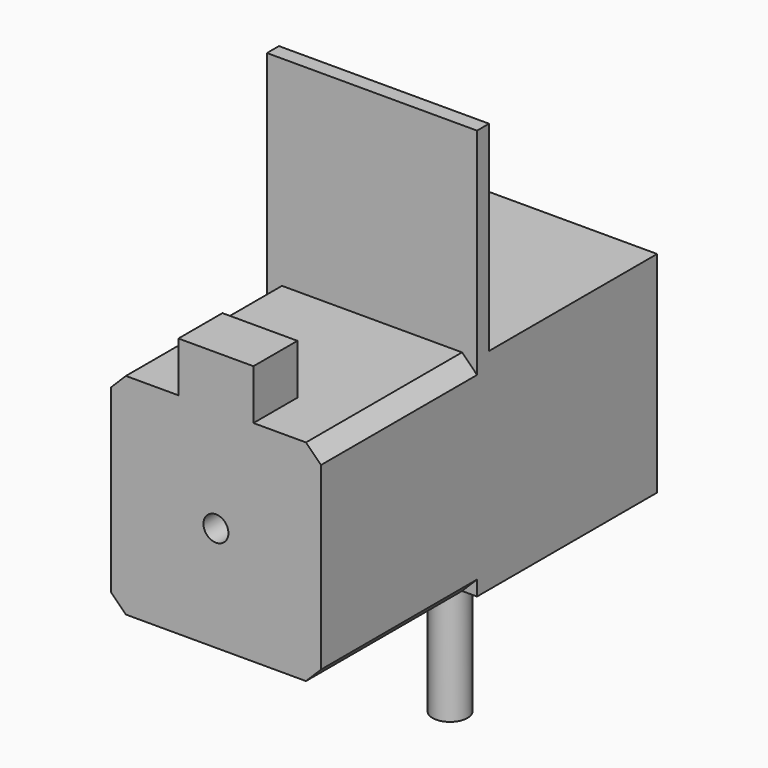
from build123d import *

# Parameters (mm, degrees)
F0_W      = 42
F0_H      = 42
F0_R      = 1.25
F0_R_2    = 11
F0_R_3    = 4.5
F0_R_4    = 2.5
F1_DEPTH  = 39
F2_SIZE   = 3
F3_DEPTH  = 2
F5_W      = 15
F5_H      = 11
F6_DEPTH  = 10
F7_DEPTH  = 45
F8_W      = 42
F8_H      = 3
F9_DEPTH  = 40
F11_DEPTH = 30


# Not quite as in the source:
# - the program builds the solid bodies; features that only make, move or delete a surface that nothing else refers to are left out


with BuildPart() as f1:
    # F0 (on Front) → F1 (new body)
    with BuildSketch(Plane.XZ):
        with Locations((-22.9883964362, 22.6771618161)):
            Rectangle(F0_W, F0_H)
        with Locations((-38.4247341791, 7.1771618161)):
            Circle(F0_R, mode=Mode.SUBTRACT)
        with Locations((-7.4883964362, 7.1771618161)):
            Circle(F0_R, mode=Mode.SUBTRACT)
        with Locations((-38.4247341791, 38.1764436699)):
            Circle(F0_R, mode=Mode.SUBTRACT)
        with Locations((-22.9883964362, 22.6771618161)):
            Circle(F0_R_2, mode=Mode.SUBTRACT)
        with Locations((-7.4883964362, 38.1778829577)):
            Circle(F0_R, mode=Mode.SUBTRACT)
        with Locations((-22.9883964362, 22.6771618161)):
            Circle(F0_R_2)
        with Locations((-22.9883964362, 22.6771618161)):
            Circle(F0_R_3, mode=Mode.SUBTRACT)
        with Locations((-22.9883964362, 22.6771618161)):
            Circle(F0_R_3)
        with Locations((-22.9883964362, 22.6771618161)):
            Circle(F0_R_4, mode=Mode.SUBTRACT)
        with Locations((-38.4247341791, 38.1764436699)):
            Circle(F0_R)
        with Locations((-7.4883964362, 7.1771618161)):
            Circle(F0_R)
        with Locations((-38.4247341791, 7.1771618161)):
            Circle(F0_R)
        with Locations((-7.4883964362, 38.1778829577)):
            Circle(F0_R)
    extrude(amount=F1_DEPTH)

    # F2
    f2_edges = [f1.edges().sort_by_distance(p)[0] for p in [
        (-43.988396, -19.5, 1.677162),
        (-1.988396, -19.5, 1.677162),
        (-1.988396, -19.5, 43.677162),
        (-43.988396, -19.5, 43.677162),
    ]]
    chamfer(f2_edges, length=F2_SIZE)

    # F0 (on Front) → F3 (join)
    with BuildSketch(Plane.XZ):
        with Locations((-22.9883964362, 22.6771618161)):
            Circle(F0_R_2)
        with Locations((-22.9883964362, 22.6771618161)):
            Circle(F0_R_3, mode=Mode.SUBTRACT)
    extrude(amount=-F3_DEPTH)

    # F5 (on face) → F6 (join)
    with BuildSketch(Plane.XY.offset(43.6771618161)):
        with Locations((-22.9883964362, -33.5)):
            Rectangle(F5_W, F5_H)
    extrude(amount=F6_DEPTH)

    # F0 (on Front) → F7 (join)
    with BuildSketch(Plane.XZ):
        with Locations((-22.9883964362, 22.6771618161)):
            Rectangle(F0_W, F0_H)
        with Locations((-38.4247341791, 7.1771618161)):
            Circle(F0_R, mode=Mode.SUBTRACT)
        with Locations((-7.4883964362, 7.1771618161)):
            Circle(F0_R, mode=Mode.SUBTRACT)
        with Locations((-38.4247341791, 38.1764436699)):
            Circle(F0_R, mode=Mode.SUBTRACT)
        with Locations((-22.9883964362, 22.6771618161)):
            Circle(F0_R_2, mode=Mode.SUBTRACT)
        with Locations((-7.4883964362, 38.1778829577)):
            Circle(F0_R, mode=Mode.SUBTRACT)
    extrude(amount=-F7_DEPTH)

    # F8 (on face) → F9 (join)
    with BuildSketch(Plane.XY.offset(43.6771618161)):
        with Locations((-22.9883964362, 1.5)):
            Rectangle(F8_W, F8_H)
    extrude(amount=F9_DEPTH)


with BuildPart() as f11:
    # F10 (on face) → F11 (new body)
    with BuildSketch(Plane(origin=(0, 0, 1.6771618161), x_dir=(1, 0, 0), z_dir=(0, 0, -1))):
        with BuildLine():
            Line((-20.4883964362, -12), (-13.4883964362, -12))
            ThreePointArc((-13.4883964362, -12), (-16.9883964362, -8.5), (-20.4883964362, -12))
        make_face()
        with BuildLine():
            ThreePointArc((-20.4883964362, -12), (-16.9883964362, -15.5), (-13.4883964362, -12))
            Line((-13.4883964362, -12), (-20.4883964362, -12))
        make_face()
    extrude(amount=F11_DEPTH)


solid = Compound([f1.part, f11.part])
